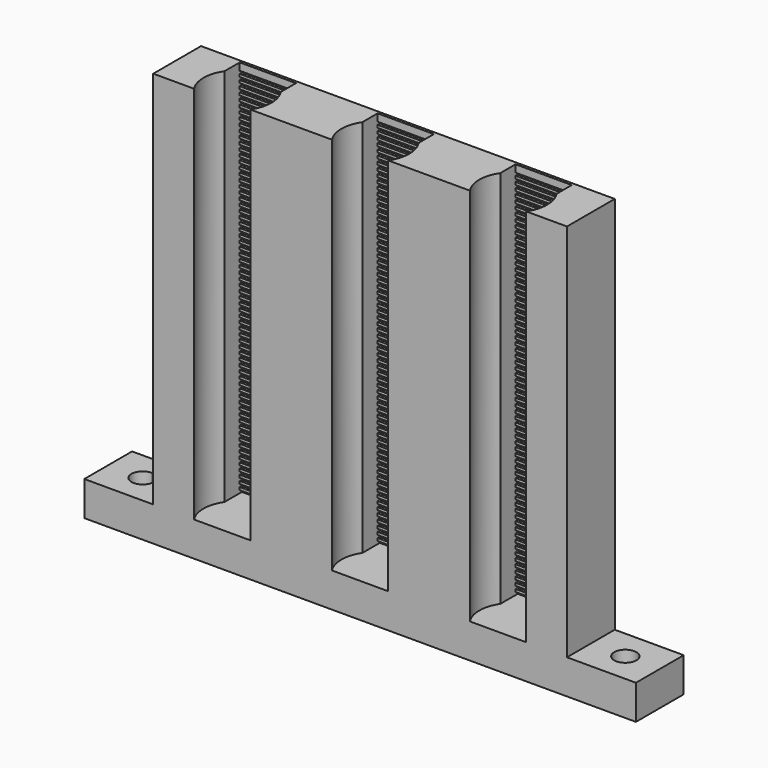
from build123d import *

# Parameters (mm, degrees)
F0_W         = 76.2
F0_H         = 11
F1_DEPTH     = 76.2
F2_R         = 6.25
F3_DEPTH     = 69.85
F4_W         = 10.3561575886
F4_H         = 0.5
F5_DEPTH     = 11
F6_TEXT_SIZE = 5.2916666667
F7_DEPTH     = 0.5
F8_W         = 10.3561575886
F8_H         = 3.5
F9_DEPTH     = 69.85
F10_W        = 11
F10_H        = 6.35
F11_DEPTH    = 12.7
F12_W        = 11
F12_H        = 6.35
F13_DEPTH    = 12.7
F14_R        = 2.05
F15_DEPTH    = 6.35


# Not quite as in the source:
# - Text() gives the source's letters only with a copy of the font that has no kerning and outlines rounded to 1/6400 em; it was checked with that copy


with BuildPart() as f1:
    # F0 (on Top) → F1 (new body)
    with BuildSketch(Plane.XY):
        Rectangle(F0_W, F0_H)
    extrude(amount=F1_DEPTH)

    # F2 (on face) → F3 (cut)
    with BuildSketch(Plane.XY.offset(76.2)):
        with BuildLine():
            ThreePointArc((0, 4.25), (-4.4194173824, -6.4194173824), (6.25, -2))
            ThreePointArc((6.25, -2), (4.4194173824, 2.4194173824), (0, 4.25))
        make_face()
        with Locations((-25.4, -2)):
            Circle(F2_R)
        with Locations((25.4, -2)):
            Circle(F2_R)
    extrude(amount=-F3_DEPTH, mode=Mode.SUBTRACT)

    # F4 (on face) → F5 (cut, through all)
    with BuildSketch(Plane(origin=(0, 5.5, 0), x_dir=(-1, 0, 0), z_dir=(0, 1, 0))):
        with Locations((-25.4, 6.6)):
            Rectangle(F4_W, F4_H)
        with Locations((-25.4, 7.6)):
            Rectangle(F4_W, F4_H)
        with Locations((-25.4, 8.6)):
            Rectangle(F4_W, F4_H)
        with Locations((-25.4, 9.6)):
            Rectangle(F4_W, F4_H)
        with Locations((-25.4, 10.6)):
            Rectangle(F4_W, F4_H)
        with Locations((-25.4, 11.6)):
            Rectangle(F4_W, F4_H)
        with Locations((-25.4, 12.6)):
            Rectangle(F4_W, F4_H)
        with Locations((-25.4, 13.6)):
            Rectangle(F4_W, F4_H)
        with Locations((-25.4, 14.6)):
            Rectangle(F4_W, F4_H)
        with Locations((-25.4, 15.6)):
            Rectangle(F4_W, F4_H)
        with Locations((-25.4, 16.6)):
            Rectangle(F4_W, F4_H)
        with Locations((-25.4, 17.6)):
            Rectangle(F4_W, F4_H)
        with Locations((-25.4, 18.6)):
            Rectangle(F4_W, F4_H)
        with Locations((-25.4, 19.6)):
            Rectangle(F4_W, F4_H)
        with Locations((-25.4, 20.6)):
            Rectangle(F4_W, F4_H)
        with Locations((-25.4, 21.6)):
            Rectangle(F4_W, F4_H)
        with Locations((0, 6.6)):
            Rectangle(F4_W, F4_H)
        with Locations((0, 7.6)):
            Rectangle(F4_W, F4_H)
        with Locations((0, 8.6)):
            Rectangle(F4_W, F4_H)
        with Locations((0, 9.6)):
            Rectangle(F4_W, F4_H)
        with Locations((0, 10.6)):
            Rectangle(F4_W, F4_H)
        with Locations((0, 11.6)):
            Rectangle(F4_W, F4_H)
        with Locations((0, 12.6)):
            Rectangle(F4_W, F4_H)
        with Locations((0, 13.6)):
            Rectangle(F4_W, F4_H)
        with Locations((0, 14.6)):
            Rectangle(F4_W, F4_H)
        with Locations((0, 15.6)):
            Rectangle(F4_W, F4_H)
        with Locations((0, 16.6)):
            Rectangle(F4_W, F4_H)
        with Locations((0, 17.6)):
            Rectangle(F4_W, F4_H)
        with Locations((0, 18.6)):
            Rectangle(F4_W, F4_H)
        with Locations((0, 19.6)):
            Rectangle(F4_W, F4_H)
        with Locations((0, 20.6)):
            Rectangle(F4_W, F4_H)
        with Locations((0, 21.6)):
            Rectangle(F4_W, F4_H)
        with Locations((25.4, 6.6)):
            Rectangle(F4_W, F4_H)
        with Locations((25.4, 7.6)):
            Rectangle(F4_W, F4_H)
        with Locations((25.4, 8.6)):
            Rectangle(F4_W, F4_H)
        with Locations((25.4, 9.6)):
            Rectangle(F4_W, F4_H)
        with Locations((25.4, 10.6)):
            Rectangle(F4_W, F4_H)
        with Locations((25.4, 11.6)):
            Rectangle(F4_W, F4_H)
        with Locations((25.4, 12.6)):
            Rectangle(F4_W, F4_H)
        with Locations((25.4, 13.6)):
            Rectangle(F4_W, F4_H)
        with Locations((25.4, 14.6)):
            Rectangle(F4_W, F4_H)
        with Locations((25.4, 15.6)):
            Rectangle(F4_W, F4_H)
        with Locations((25.4, 16.6)):
            Rectangle(F4_W, F4_H)
        with Locations((25.4, 17.6)):
            Rectangle(F4_W, F4_H)
        with Locations((25.4, 18.6)):
            Rectangle(F4_W, F4_H)
        with Locations((25.4, 19.6)):
            Rectangle(F4_W, F4_H)
        with Locations((25.4, 20.6)):
            Rectangle(F4_W, F4_H)
        with Locations((25.4, 21.6)):
            Rectangle(F4_W, F4_H)
        with Locations((-25.4, 22.6)):
            Rectangle(F4_W, F4_H)
        with Locations((-25.4, 23.6)):
            Rectangle(F4_W, F4_H)
        with Locations((0, 22.6)):
            Rectangle(F4_W, F4_H)
        with Locations((0, 23.6)):
            Rectangle(F4_W, F4_H)
        with Locations((25.4, 22.6)):
            Rectangle(F4_W, F4_H)
        with Locations((25.4, 23.6)):
            Rectangle(F4_W, F4_H)
        with Locations((-25.4, 24.6)):
            Rectangle(F4_W, F4_H)
        with Locations((-25.4, 25.6)):
            Rectangle(F4_W, F4_H)
        with Locations((-25.4, 26.6)):
            Rectangle(F4_W, F4_H)
        with Locations((-25.4, 27.6)):
            Rectangle(F4_W, F4_H)
        with Locations((-25.4, 28.6)):
            Rectangle(F4_W, F4_H)
        with Locations((-25.4, 29.6)):
            Rectangle(F4_W, F4_H)
        with Locations((-25.4, 30.6)):
            Rectangle(F4_W, F4_H)
        with Locations((-25.4, 31.6)):
            Rectangle(F4_W, F4_H)
        with Locations((-25.4, 32.6)):
            Rectangle(F4_W, F4_H)
        with Locations((-25.4, 33.6)):
            Rectangle(F4_W, F4_H)
        with Locations((-25.4, 34.6)):
            Rectangle(F4_W, F4_H)
        with Locations((-25.4, 35.6)):
            Rectangle(F4_W, F4_H)
        with Locations((-25.4, 36.6)):
            Rectangle(F4_W, F4_H)
        with Locations((-25.4, 37.6)):
            Rectangle(F4_W, F4_H)
        with Locations((-25.4, 38.6)):
            Rectangle(F4_W, F4_H)
        with Locations((-25.4, 39.6)):
            Rectangle(F4_W, F4_H)
        with Locations((-25.4, 40.6)):
            Rectangle(F4_W, F4_H)
        with Locations((-25.4, 41.6)):
            Rectangle(F4_W, F4_H)
        with Locations((-25.4, 42.6)):
            Rectangle(F4_W, F4_H)
        with Locations((-25.4, 43.6)):
            Rectangle(F4_W, F4_H)
        with Locations((-25.4, 44.6)):
            Rectangle(F4_W, F4_H)
        with Locations((-25.4, 45.6)):
            Rectangle(F4_W, F4_H)
        with Locations((-25.4, 46.6)):
            Rectangle(F4_W, F4_H)
        with Locations((-25.4, 47.6)):
            Rectangle(F4_W, F4_H)
        with Locations((-25.4, 48.6)):
            Rectangle(F4_W, F4_H)
        with Locations((-25.4, 49.6)):
            Rectangle(F4_W, F4_H)
        with Locations((-25.4, 50.6)):
            Rectangle(F4_W, F4_H)
        with Locations((-25.4, 51.6)):
            Rectangle(F4_W, F4_H)
        with Locations((-25.4, 52.6)):
            Rectangle(F4_W, F4_H)
        with Locations((-25.4, 53.6)):
            Rectangle(F4_W, F4_H)
        with Locations((-25.4, 54.6)):
            Rectangle(F4_W, F4_H)
        with Locations((-25.4, 55.6)):
            Rectangle(F4_W, F4_H)
        with Locations((-25.4, 56.6)):
            Rectangle(F4_W, F4_H)
        with Locations((-25.4, 57.6)):
            Rectangle(F4_W, F4_H)
        with Locations((-25.4, 58.6)):
            Rectangle(F4_W, F4_H)
        with Locations((-25.4, 59.6)):
            Rectangle(F4_W, F4_H)
        with Locations((-25.4, 60.6)):
            Rectangle(F4_W, F4_H)
        with Locations((-25.4, 61.6)):
            Rectangle(F4_W, F4_H)
        with Locations((-25.4, 62.6)):
            Rectangle(F4_W, F4_H)
        with Locations((-25.4, 63.6)):
            Rectangle(F4_W, F4_H)
        with Locations((-25.4, 64.6)):
            Rectangle(F4_W, F4_H)
        with Locations((-25.4, 65.6)):
            Rectangle(F4_W, F4_H)
        with Locations((-25.4, 66.6)):
            Rectangle(F4_W, F4_H)
        with Locations((-25.4, 67.6)):
            Rectangle(F4_W, F4_H)
        with Locations((-25.4, 68.6)):
            Rectangle(F4_W, F4_H)
        with Locations((-25.4, 69.6)):
            Rectangle(F4_W, F4_H)
        with Locations((-25.4, 70.6)):
            Rectangle(F4_W, F4_H)
        with Locations((-25.4, 71.6)):
            Rectangle(F4_W, F4_H)
        with Locations((-25.4, 72.6)):
            Rectangle(F4_W, F4_H)
        with Locations((-25.4, 73.6)):
            Rectangle(F4_W, F4_H)
        with Locations((-25.4, 74.6)):
            Rectangle(F4_W, F4_H)
        with Locations((0, 24.6)):
            Rectangle(F4_W, F4_H)
        with Locations((0, 25.6)):
            Rectangle(F4_W, F4_H)
        with Locations((0, 26.6)):
            Rectangle(F4_W, F4_H)
        with Locations((0, 27.6)):
            Rectangle(F4_W, F4_H)
        with Locations((0, 28.6)):
            Rectangle(F4_W, F4_H)
        with Locations((0, 29.6)):
            Rectangle(F4_W, F4_H)
        with Locations((0, 30.6)):
            Rectangle(F4_W, F4_H)
        with Locations((0, 31.6)):
            Rectangle(F4_W, F4_H)
        with Locations((0, 32.6)):
            Rectangle(F4_W, F4_H)
        with Locations((0, 33.6)):
            Rectangle(F4_W, F4_H)
        with Locations((0, 34.6)):
            Rectangle(F4_W, F4_H)
        with Locations((0, 35.6)):
            Rectangle(F4_W, F4_H)
        with Locations((0, 36.6)):
            Rectangle(F4_W, F4_H)
        with Locations((0, 37.6)):
            Rectangle(F4_W, F4_H)
        with Locations((0, 38.6)):
            Rectangle(F4_W, F4_H)
        with Locations((0, 39.6)):
            Rectangle(F4_W, F4_H)
        with Locations((0, 40.6)):
            Rectangle(F4_W, F4_H)
        with Locations((0, 41.6)):
            Rectangle(F4_W, F4_H)
        with Locations((0, 42.6)):
            Rectangle(F4_W, F4_H)
        with Locations((0, 43.6)):
            Rectangle(F4_W, F4_H)
        with Locations((0, 44.6)):
            Rectangle(F4_W, F4_H)
        with Locations((0, 45.6)):
            Rectangle(F4_W, F4_H)
        with Locations((0, 46.6)):
            Rectangle(F4_W, F4_H)
        with Locations((0, 47.6)):
            Rectangle(F4_W, F4_H)
        with Locations((0, 48.6)):
            Rectangle(F4_W, F4_H)
        with Locations((0, 49.6)):
            Rectangle(F4_W, F4_H)
        with Locations((0, 50.6)):
            Rectangle(F4_W, F4_H)
        with Locations((0, 51.6)):
            Rectangle(F4_W, F4_H)
        with Locations((0, 52.6)):
            Rectangle(F4_W, F4_H)
        with Locations((0, 53.6)):
            Rectangle(F4_W, F4_H)
        with Locations((0, 54.6)):
            Rectangle(F4_W, F4_H)
        with Locations((0, 55.6)):
            Rectangle(F4_W, F4_H)
        with Locations((0, 56.6)):
            Rectangle(F4_W, F4_H)
        with Locations((0, 57.6)):
            Rectangle(F4_W, F4_H)
        with Locations((0, 58.6)):
            Rectangle(F4_W, F4_H)
        with Locations((0, 59.6)):
            Rectangle(F4_W, F4_H)
        with Locations((0, 60.6)):
            Rectangle(F4_W, F4_H)
        with Locations((0, 61.6)):
            Rectangle(F4_W, F4_H)
        with Locations((0, 62.6)):
            Rectangle(F4_W, F4_H)
        with Locations((0, 63.6)):
            Rectangle(F4_W, F4_H)
        with Locations((0, 64.6)):
            Rectangle(F4_W, F4_H)
        with Locations((0, 65.6)):
            Rectangle(F4_W, F4_H)
        with Locations((0, 66.6)):
            Rectangle(F4_W, F4_H)
        with Locations((0, 67.6)):
            Rectangle(F4_W, F4_H)
        with Locations((0, 68.6)):
            Rectangle(F4_W, F4_H)
        with Locations((0, 69.6)):
            Rectangle(F4_W, F4_H)
        with Locations((0, 70.6)):
            Rectangle(F4_W, F4_H)
        with Locations((0, 71.6)):
            Rectangle(F4_W, F4_H)
        with Locations((0, 72.6)):
            Rectangle(F4_W, F4_H)
        with Locations((0, 73.6)):
            Rectangle(F4_W, F4_H)
        with Locations((0, 74.6)):
            Rectangle(F4_W, F4_H)
        with Locations((25.4, 24.6)):
            Rectangle(F4_W, F4_H)
        with Locations((25.4, 25.6)):
            Rectangle(F4_W, F4_H)
        with Locations((25.4, 26.6)):
            Rectangle(F4_W, F4_H)
        with Locations((25.4, 27.6)):
            Rectangle(F4_W, F4_H)
        with Locations((25.4, 28.6)):
            Rectangle(F4_W, F4_H)
        with Locations((25.4, 29.6)):
            Rectangle(F4_W, F4_H)
        with Locations((25.4, 30.6)):
            Rectangle(F4_W, F4_H)
        with Locations((25.4, 31.6)):
            Rectangle(F4_W, F4_H)
        with Locations((25.4, 32.6)):
            Rectangle(F4_W, F4_H)
        with Locations((25.4, 33.6)):
            Rectangle(F4_W, F4_H)
        with Locations((25.4, 34.6)):
            Rectangle(F4_W, F4_H)
        with Locations((25.4, 35.6)):
            Rectangle(F4_W, F4_H)
        with Locations((25.4, 36.6)):
            Rectangle(F4_W, F4_H)
        with Locations((25.4, 37.6)):
            Rectangle(F4_W, F4_H)
        with Locations((25.4, 38.6)):
            Rectangle(F4_W, F4_H)
        with Locations((25.4, 39.6)):
            Rectangle(F4_W, F4_H)
        with Locations((25.4, 40.6)):
            Rectangle(F4_W, F4_H)
        with Locations((25.4, 41.6)):
            Rectangle(F4_W, F4_H)
        with Locations((25.4, 42.6)):
            Rectangle(F4_W, F4_H)
        with Locations((25.4, 43.6)):
            Rectangle(F4_W, F4_H)
        with Locations((25.4, 44.6)):
            Rectangle(F4_W, F4_H)
        with Locations((25.4, 45.6)):
            Rectangle(F4_W, F4_H)
        with Locations((25.4, 46.6)):
            Rectangle(F4_W, F4_H)
        with Locations((25.4, 47.6)):
            Rectangle(F4_W, F4_H)
        with Locations((25.4, 48.6)):
            Rectangle(F4_W, F4_H)
        with Locations((25.4, 49.6)):
            Rectangle(F4_W, F4_H)
        with Locations((25.4, 50.6)):
            Rectangle(F4_W, F4_H)
        with Locations((25.4, 51.6)):
            Rectangle(F4_W, F4_H)
        with Locations((25.4, 52.6)):
            Rectangle(F4_W, F4_H)
        with Locations((25.4, 53.6)):
            Rectangle(F4_W, F4_H)
        with Locations((25.4, 54.6)):
            Rectangle(F4_W, F4_H)
        with Locations((25.4, 55.6)):
            Rectangle(F4_W, F4_H)
        with Locations((25.4, 56.6)):
            Rectangle(F4_W, F4_H)
        with Locations((25.4, 57.6)):
            Rectangle(F4_W, F4_H)
        with Locations((25.4, 58.6)):
            Rectangle(F4_W, F4_H)
        with Locations((25.4, 59.6)):
            Rectangle(F4_W, F4_H)
        with Locations((25.4, 60.6)):
            Rectangle(F4_W, F4_H)
        with Locations((25.4, 61.6)):
            Rectangle(F4_W, F4_H)
        with Locations((25.4, 62.6)):
            Rectangle(F4_W, F4_H)
        with Locations((25.4, 63.6)):
            Rectangle(F4_W, F4_H)
        with Locations((25.4, 64.6)):
            Rectangle(F4_W, F4_H)
        with Locations((25.4, 65.6)):
            Rectangle(F4_W, F4_H)
        with Locations((25.4, 66.6)):
            Rectangle(F4_W, F4_H)
        with Locations((25.4, 67.6)):
            Rectangle(F4_W, F4_H)
        with Locations((25.4, 68.6)):
            Rectangle(F4_W, F4_H)
        with Locations((25.4, 69.6)):
            Rectangle(F4_W, F4_H)
        with Locations((25.4, 70.6)):
            Rectangle(F4_W, F4_H)
        with Locations((25.4, 71.6)):
            Rectangle(F4_W, F4_H)
        with Locations((25.4, 72.6)):
            Rectangle(F4_W, F4_H)
        with Locations((25.4, 73.6)):
            Rectangle(F4_W, F4_H)
        with Locations((25.4, 74.6)):
            Rectangle(F4_W, F4_H)
    extrude(amount=-F5_DEPTH, mode=Mode.SUBTRACT)

    # F6 (on face) → F7 (cut)
    with BuildSketch(Plane(origin=(0, 5.5, 0), x_dir=(-1, 0, 0), z_dir=(0, 1, 0))):
        with Locations((-26.8469244572, 1.5566079867)):
            Text('1', F6_TEXT_SIZE, font='Open Sans', text_align=(TextAlign.LEFT, TextAlign.BOTTOM))
        with Locations((-1.5416732874, 1.5566079867)):
            Text('2', F6_TEXT_SIZE, font='Open Sans', text_align=(TextAlign.LEFT, TextAlign.BOTTOM))
        with Locations((24.0893187388, 1.5566079867)):
            Text('3', F6_TEXT_SIZE, font='Open Sans', text_align=(TextAlign.LEFT, TextAlign.BOTTOM))
    extrude(amount=-F7_DEPTH, mode=Mode.SUBTRACT)

    # F8 (on face) → F9 (cut, through all)
    with BuildSketch(Plane.XY.offset(76.2)):
        with Locations((25.4, 3.25)):
            Rectangle(F8_W, F8_H)
        with Locations((0, 3.25)):
            Rectangle(F8_W, F8_H)
        with Locations((-25.4, 3.25)):
            Rectangle(F8_W, F8_H)
    extrude(amount=-F9_DEPTH, mode=Mode.SUBTRACT)

    # F10 (on face) → F11 (join)
    with BuildSketch(Plane.YZ.offset(38.1)):
        with Locations((0, 3.175)):
            Rectangle(F10_W, F10_H)
    extrude(amount=F11_DEPTH)

    # F12 (on face) → F13 (join)
    with BuildSketch(Plane(origin=(-38.1, 0, 0), x_dir=(0, -1, 0), z_dir=(-1, 0, 0))):
        with Locations((0, 3.175)):
            Rectangle(F12_W, F12_H)
    extrude(amount=F13_DEPTH)

    # F14 (on face) → F15 (cut, through all)
    with BuildSketch(Plane.XY.offset(6.35)):
        with BuildLine():
            ThreePointArc((-44.45, -2.05), (-43.0004310986, -1.4495689014), (-42.4, 0))
            ThreePointArc((-42.4, 0), (-43.0004310986, 1.4495689014), (-44.45, 2.05))
            Line((-44.45, 2.05), (-44.45, -2.05))
        make_face()
        with BuildLine():
            Line((-44.45, -2.05), (-44.45, 2.05))
            ThreePointArc((-44.45, 2.05), (-46.5, 0), (-44.45, -2.05))
        make_face()
        with Locations((44.45, 0)):
            Circle(F14_R)
    extrude(amount=-F15_DEPTH, mode=Mode.SUBTRACT)


solid = f1.part
